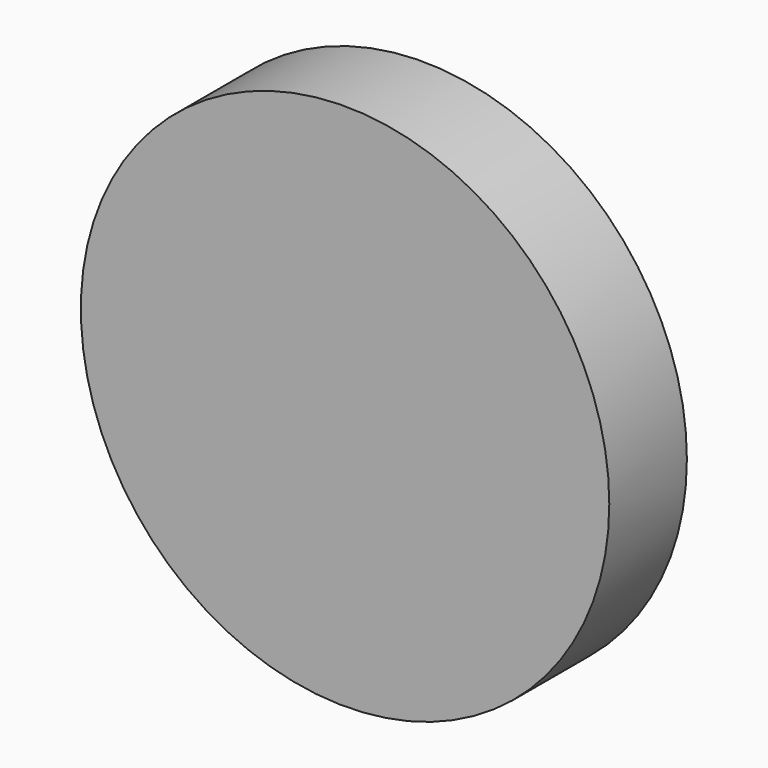
from build123d import *

# Parameters (mm, degrees)
F0_R     = 40.861011546
F1_DEPTH = 15


# Not quite as in the source:
# - a feature of the source that left no trace in its solid (it failed there, or was rolled back) is left out


with BuildPart() as f1:
    # F0 (on Front) → F1 (new body)
    with BuildSketch(Plane.XZ):
        Circle(F0_R)
    extrude(amount=F1_DEPTH)


solid = f1.part
